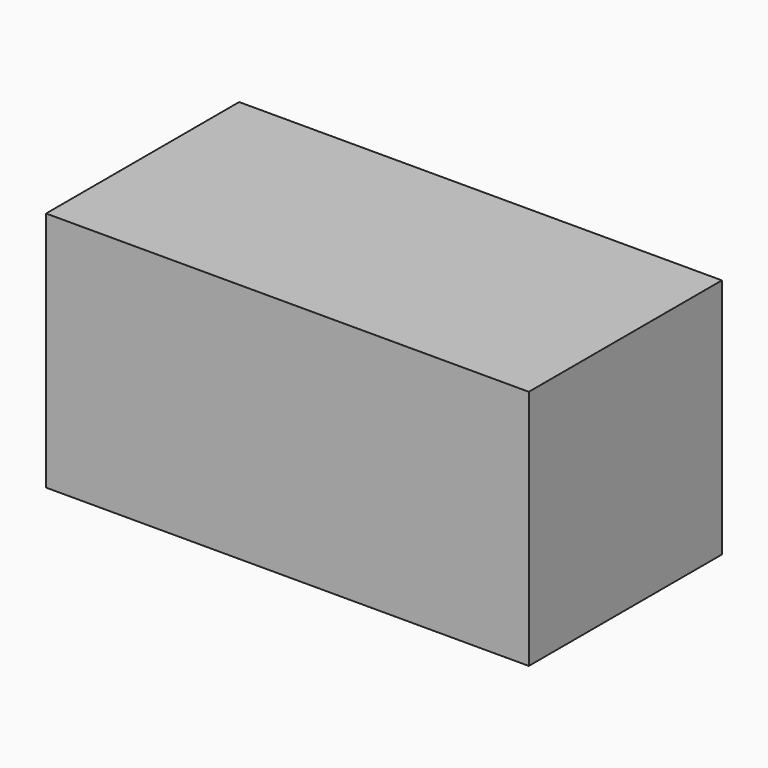
from build123d import *

# Parameters (mm, degrees)
F0_W        = 50800
F0_H        = 25400
F1_DEPTH    = 25400
F2_R        = 5.08
F3_T1_DEPTH = 25420.32
F3_T3_DEPTH = 50825.4


# Not quite as in the source:
# - a fillet or chamfer that OpenCascade refuses, or shapes differently, is made with other operations: its cross-section is extruded or revolved along the edge and cut away or added


with BuildPart() as f1:
    # F0 (on Front) → F1 (new body)
    with BuildSketch(Plane.XZ):
        with Locations((-25400, 12700)):
            Rectangle(F0_W, F0_H)
    extrude(amount=F1_DEPTH)

    # F2
    f2_edges = [f1.edges().sort_by_distance(p)[0] for p in [
        (0, -12700, 25400),
        (-50800, -12700, 25400),
        (-25400, 0, 25400),
        (-25400, -25400, 25400),
        (-25400, -25400, 0),
        (0, -25400, 12700),
        (-50800, -25400, 12700),
    ]]
    fillet(f2_edges, radius=F2_R)

    # F3: fillet of radius 5.08 on 8 edges, made by hand

    # F3_s2 → F3_t1 (cut)
    with BuildSketch(Plane.XZ.offset(-12.7)):
        with BuildLine():
            ThreePointArc((-50794.92, 0), (-50798.5121024484, 1.4878975516), (-50800, 5.08))
            Line((-50800, 5.08), (-50800, 0))
            Line((-50800, 0), (-50794.92, 0))
        make_face()
        with BuildLine():
            ThreePointArc((-5.08, 0), (-1.4878975516, 1.4878975516), (0, 5.08))
            Line((0, 5.08), (0, 0))
            Line((0, 0), (-5.08, 0))
        make_face()
    extrude(amount=F3_T1_DEPTH, mode=Mode.SUBTRACT)

    # F3_s4 → F3_t3 (cut)
    with BuildSketch(Plane.YZ.offset(-50812.7)):
        with BuildLine():
            ThreePointArc((-5.08, 0), (-1.4878975516, 1.4878975516), (0, 5.08))
            Line((0, 5.08), (0, 0))
            Line((0, 0), (-5.08, 0))
        make_face()
    extrude(amount=F3_T3_DEPTH, mode=Mode.SUBTRACT)


solid = f1.part
